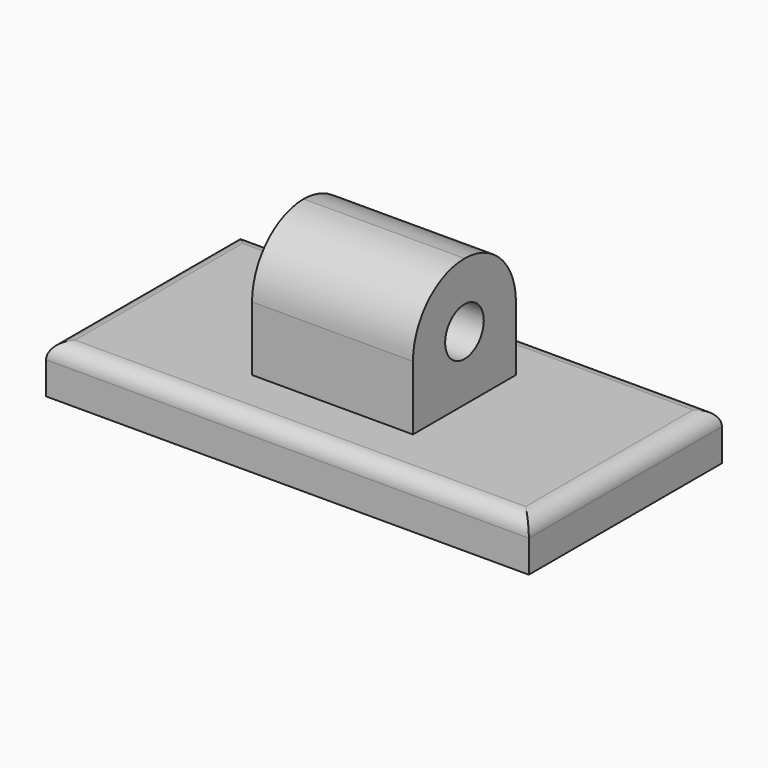
from build123d import *

# Parameters (mm, degrees)
F0_W     = 30
F0_H     = 15
F1_DEPTH = 3
F2_W     = 10
F2_H     = 8
F3_DEPTH = 8
F4_R     = 3.99999
F5_R     = 1.5
F6_DEPTH = 25
F7_R     = 1
F8_R     = 2.5
F9_DEPTH = 3
F10_R    = 0.2


# Not quite as in the source:
# - a fillet or chamfer is up to 0.001 mm smaller than in the source, because OpenCascade refuses the exact size


with BuildPart() as f1:
    # F0 (on Top) → F1 (new body)
    with BuildSketch(Plane.XY):
        with Locations((-8.5063918959, 3.0821188468)):
            Rectangle(F0_W, F0_H)
    extrude(amount=F1_DEPTH)

    # F2 (on face) → F3 (join)
    with BuildSketch(Plane.XY.offset(3)):
        with Locations((-8.5063918959, 3.0821188468)):
            Rectangle(F2_W, F2_H)
    extrude(amount=F3_DEPTH)

    # F4 (radius 4 in the source; OpenCascade refuses exactly that, so slightly less here)
    f4_edges = [f1.edges().sort_by_distance(p)[0] for p in [
        (-8.506392, -0.917881, 11),
        (-8.506392, 7.082119, 11),
    ]]
    fillet(f4_edges, radius=F4_R)

    # F5 (on face) → F6 (cut)
    with BuildSketch(Plane.YZ.offset(-3.5063918959)):
        with Locations((3.0821188468, 7)):
            Circle(F5_R)
    extrude(amount=-F6_DEPTH, mode=Mode.SUBTRACT)

    # F7
    f7_edges = [f1.edges().sort_by_distance(p)[0] for p in [
        (-23.506392, 3.082119, 3),
        (-8.506392, 10.582119, 3),
        (6.493608, 3.082119, 3),
        (-8.506392, -4.417881, 3),
    ]]
    fillet(f7_edges, radius=F7_R)

    # F8 (on face) → F9 (join)
    with BuildSketch(Plane(origin=(0, 0, 0), x_dir=(1, 0, 0), z_dir=(0, 0, -1))):
        with Locations((-16.0063918959, -3.0821188468)):
            Circle(F8_R)
        with Locations((-1.0063918959, -3.0821188468)):
            Circle(F8_R)
    extrude(amount=F9_DEPTH)

    # F10
    f10_edges = [f1.edges().sort_by_distance(p)[0] for p in [
        (-18.506392, 3.082119, -3),
        (-3.506392, 3.082119, -3),
    ]]
    fillet(f10_edges, radius=F10_R)


solid = f1.part
